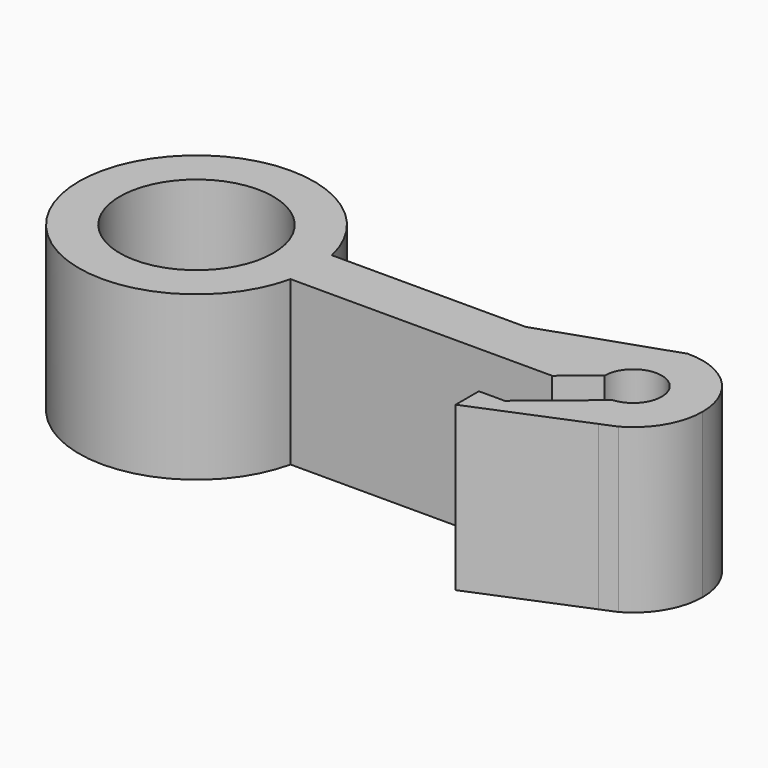
from build123d import *

# Parameters (mm, degrees)
F1_DEPTH = 10
F2_R     = 1


# Not quite as in the source:
# - a feature names something its author has since deleted; it is built from what else it names


with BuildPart() as f1:
    # F0 (on Top) → F1 (new body)
    with BuildSketch(Plane.XY):
        with BuildLine():
            ThreePointArc((-4.4255569592, 1.5825440281), (0, 4.7), (4.4255569592, 1.5825440281))
            Line((4.4255569592, 1.5825440281), (7.0239272775, 1.5825440281))
            ThreePointArc((7.0239272775, 1.5825440281), (0, 7.2), (-7.0239272775, 1.5825440281))
            Line((-7.0239272775, 1.5825440281), (-4.4255569592, 1.5825440281))
        make_face()
        with BuildLine():
            ThreePointArc((-4.4255569592, -1.5825440281), (-4.7, 0), (-4.4255569592, 1.5825440281))
            Line((-4.4255569592, 1.5825440281), (-7.0239272775, 1.5825440281))
            ThreePointArc((-7.0239272775, 1.5825440281), (-7.2, 0), (-7.0239272775, -1.5825440281))
            Line((-7.0239272775, -1.5825440281), (-4.4255569592, -1.5825440281))
        make_face()
        with BuildLine():
            Line((7.0239272775, -1.5825440281), (4.4255569592, -1.5825440281))
            ThreePointArc((4.4255569592, -1.5825440281), (0, -4.7), (-4.4255569592, -1.5825440281))
            Line((-4.4255569592, -1.5825440281), (-7.0239272775, -1.5825440281))
            ThreePointArc((-7.0239272775, -1.5825440281), (0, -7.2), (7.0239272775, -1.5825440281))
        make_face()
        with BuildLine():
            ThreePointArc((4.4255569592, 1.5825440281), (4.6308810019, 0.8030822784), (4.7, 0))
            ThreePointArc((4.7, 0), (4.6308810019, -0.8030822784), (4.4255569592, -1.5825440281))
            Line((4.4255569592, -1.5825440281), (7.0239272775, -1.5825440281))
            ThreePointArc((7.0239272775, -1.5825440281), (7.1558464348, -0.7961543827), (7.2, 0))
            ThreePointArc((7.2, 0), (7.1558464348, 0.7961543827), (7.0239272775, 1.5825440281))
            Line((7.0239272775, 1.5825440281), (4.4255569592, 1.5825440281))
        make_face()
        with BuildLine():
            ThreePointArc((24.1954502469, 3.3965829239), (23.3763263872, 2.5847294548), (22.8056300377, 1.5825440281))
            Line((22.8056300377, 1.5825440281), (25, 1.5825440281))
            Line((25, 1.5825440281), (25, 0))
            ThreePointArc((25, 0), (26.75, 1.75), (28.5, 0))
            ThreePointArc((28.5, 0), (28.0337651782, -1.1893052456), (26.8834891802, -1.7449013264))
            Line((26.8834891802, -1.7449013264), (24.5703446749, -3.6485069089))
            ThreePointArc((24.5703446749, -3.6485069089), (26.1897753497, -4.2129144711), (27.9004272408, -4.0913343989))
            Line((27.9004272408, -4.0913343989), (28.8181424703, -3.7128542555))
            ThreePointArc((28.8181424703, -3.7128542555), (30.41415785, -2.1532411037), (31, 0))
            ThreePointArc((31, 0), (29.7329020897, 3.0273412631), (26.6871552362, 4.2495353317))
            Line((26.6871552362, 4.2495353317), (24.1954502469, 3.3965829239))
        make_face()
        with BuildLine():
            ThreePointArc((22.8056300377, 1.5825440281), (22.5, 0), (22.8056300377, -1.5825440281))
            Line((22.8056300377, -1.5825440281), (23.0520843585, -1.5825440281))
            Line((23.0520843585, -1.5825440281), (25, 0))
            Line((25, 0), (25, 1.5825440281))
            Line((25, 1.5825440281), (22.8056300377, 1.5825440281))
        make_face()
        with BuildLine():
            Line((18.896151334, 1.5825440281), (7.0239272775, 1.5825440281))
            ThreePointArc((7.0239272775, 1.5825440281), (7.1558464348, 0.7961543827), (7.2, 0))
            ThreePointArc((7.2, 0), (7.1558464348, -0.7961543827), (7.0239272775, -1.5825440281))
            Line((7.0239272775, -1.5825440281), (22.8056300377, -1.5825440281))
            ThreePointArc((22.8056300377, -1.5825440281), (22.5, 0), (22.8056300377, 1.5825440281))
            Line((22.8056300377, 1.5825440281), (18.896151334, 1.5825440281))
        make_face()
        with BuildLine():
            Line((24.1954502469, 3.3965829239), (18.896151334, 1.5825440281))
            Line((18.896151334, 1.5825440281), (22.8056300377, 1.5825440281))
            ThreePointArc((22.8056300377, 1.5825440281), (23.3763263872, 2.5847294548), (24.1954502469, 3.3965829239))
        make_face()
        with BuildLine():
            ThreePointArc((27.9004272408, -4.0913343989), (26.1897753497, -4.2129144711), (24.5703446749, -3.6485069089))
            Line((24.5703446749, -3.6485069089), (22.897355554, -5.0252957012))
            Line((22.897355554, -5.0252957012), (21.3165715317, -5.0252957012))
            Line((21.3165715317, -5.0252957012), (21.3165715317, -6.8066196779))
            Line((21.3165715317, -6.8066196779), (27.9004272408, -4.0913343989))
        make_face()
    extrude(amount=F1_DEPTH)

    # F2
    f2_edges = [f1.edges().sort_by_distance(p)[0] for p in [
        (-4.425557, -1.582544, 0),
    ]]
    fillet(f2_edges, radius=F2_R)


solid = f1.part
